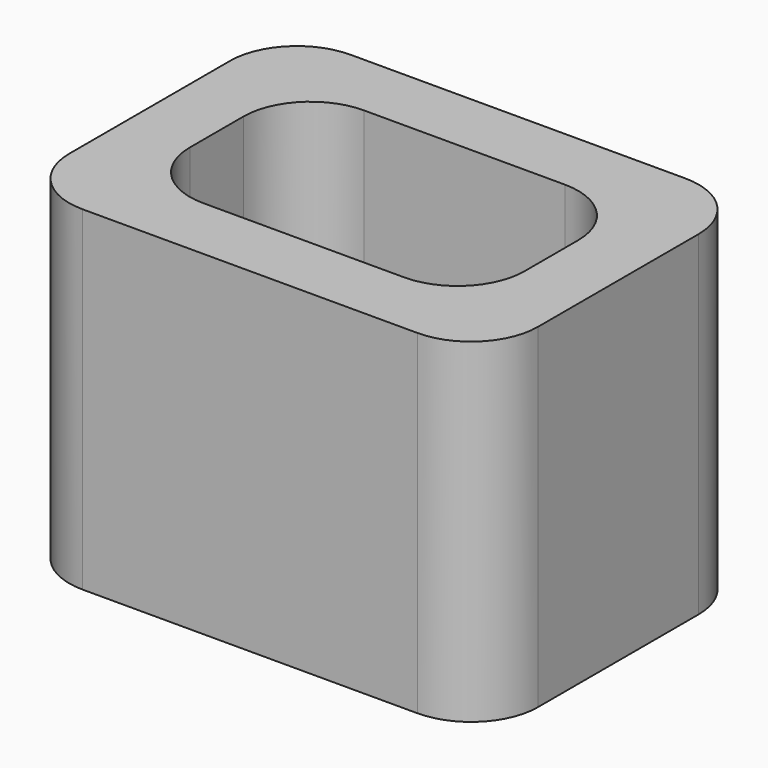
from build123d import *

# Parameters (mm, degrees)
F0_W        = 177.8
F0_H        = 127
F1_DEPTH    = 127
F2_R        = 25.4
F3_T        = 25.4
F4_T1_DEPTH = 101.6


# Not quite as in the source:
# - a fillet or chamfer that OpenCascade refuses, or shapes differently, is made with other operations: its cross-section is extruded or revolved along the edge and cut away or added
# - a shell that OpenCascade refuses in one call is made with other operations: the cavity is built on its own and cut out


with BuildPart() as f1:
    # F0 (on Top) → F1 (new body)
    with BuildSketch(Plane.XY):
        with Locations((88.9, -63.5)):
            Rectangle(F0_W, F0_H)
    extrude(amount=F1_DEPTH)

    # F2
    f2_edges = [f1.edges().sort_by_distance(p)[0] for p in [
        (0, -127, 63.5),
        (177.8, -127, 63.5),
        (177.8, 0, 63.5),
        (0, 0, 63.5),
    ]]
    fillet(f2_edges, radius=F2_R)

    # F3: shell of thickness 25.4, made by hand


with BuildPart() as f3_core1:
    # F3_t2: copy of F1
    add(f1.part)

    # the walls: a layer under each face that stays
    f3_faces = [f3_core1.faces().sort_by_distance(p)[0] for p in [
        (88.9, 0, 63.5),
        (88.9, -63.5, 0),
        (177.8, -63.5, 63.5),
        (0, -63.5, 63.5),
        (88.9, -127, 63.5),
    ]]
    thicken(f3_faces, amount=-F3_T, mode=Mode.SUBTRACT)


with BuildPart() as f1_1:
    add(f1.part)

    # what is left inside the walls is the cavity
    f3_cavity = [f3_core1.part.solids().sort_by_distance(p)[0] for p in [
        (88.9, -25.654, 93.133333),
    ]]
    add(f3_cavity, mode=Mode.SUBTRACT)

    # F4: fillet of radius 25.4 on 6 edges, made by hand

    # F4_s2 → F4_t1 (join)
    with BuildSketch(Plane.XY.offset(25.4)):
        with BuildLine():
            ThreePointArc((50.8, -25.4), (32.8394877579, -32.8394877579), (25.4, -50.8))
            Line((25.4, -50.8), (25.4, -25.4))
            Line((25.4, -25.4), (50.8, -25.4))
        make_face()
        with BuildLine():
            ThreePointArc((127, -25.4), (144.9605122421, -32.8394877579), (152.4, -50.8))
            Line((152.4, -50.8), (152.4, -25.4))
            Line((152.4, -25.4), (127, -25.4))
        make_face()
        with BuildLine():
            ThreePointArc((25.4, -76.2), (32.8394877579, -94.1605122421), (50.8, -101.6))
            Line((50.8, -101.6), (25.4, -101.6))
            Line((25.4, -101.6), (25.4, -76.2))
        make_face()
        with BuildLine():
            ThreePointArc((127, -101.6), (144.9605122421, -94.1605122421), (152.4, -76.2))
            Line((152.4, -76.2), (152.4, -101.6))
            Line((152.4, -101.6), (127, -101.6))
        make_face()
    extrude(amount=F4_T1_DEPTH)


solid = f1_1.part
